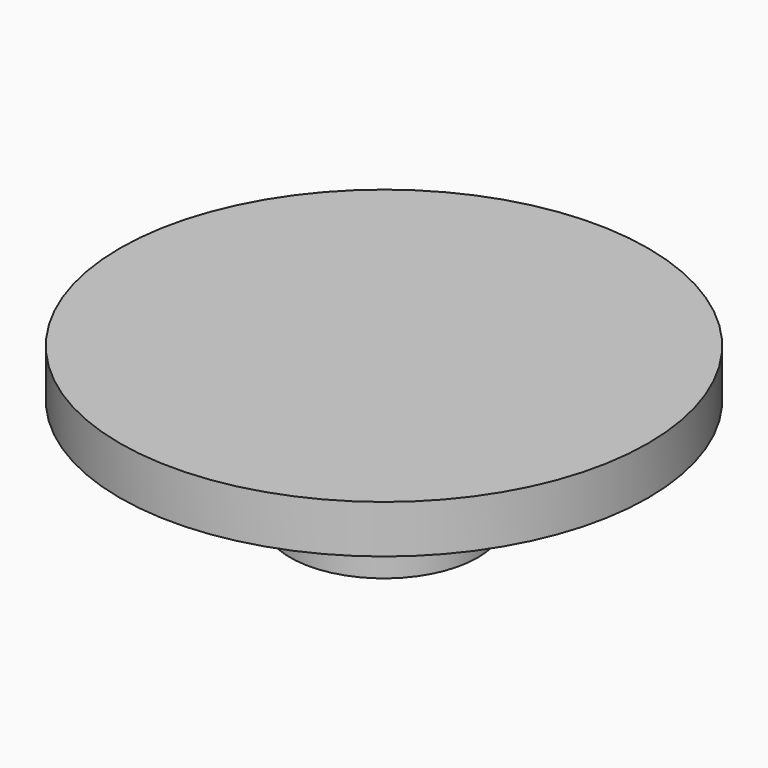
from build123d import *

# Parameters (mm, degrees)
F1_START = 4.5
F0_R     = 11
F1_DEPTH = 2
F2_R     = 3.9
F2_R_2   = 2.5
F3_DEPTH = 3.5
F5_START = 3.5
F4_R     = 5.75
F5_DEPTH = 1


with BuildPart() as f1:
    # F0 (on Top) → F1 (new body)
    with BuildSketch(Plane.XY.offset(F1_START)):
        Circle(F0_R)
    extrude(amount=F1_DEPTH)


with BuildPart() as f3:
    # F2 (on Top) → F3 (new body)
    with BuildSketch(Plane.XY):
        Circle(F2_R)
        Circle(F2_R_2, mode=Mode.SUBTRACT)
    extrude(amount=F3_DEPTH)

    # F4 (on Top) → F5 (join)
    with BuildSketch(Plane.XY.offset(F5_START)):
        Circle(F4_R)
    extrude(amount=F5_DEPTH)


solid = Compound([f1.part, f3.part])
